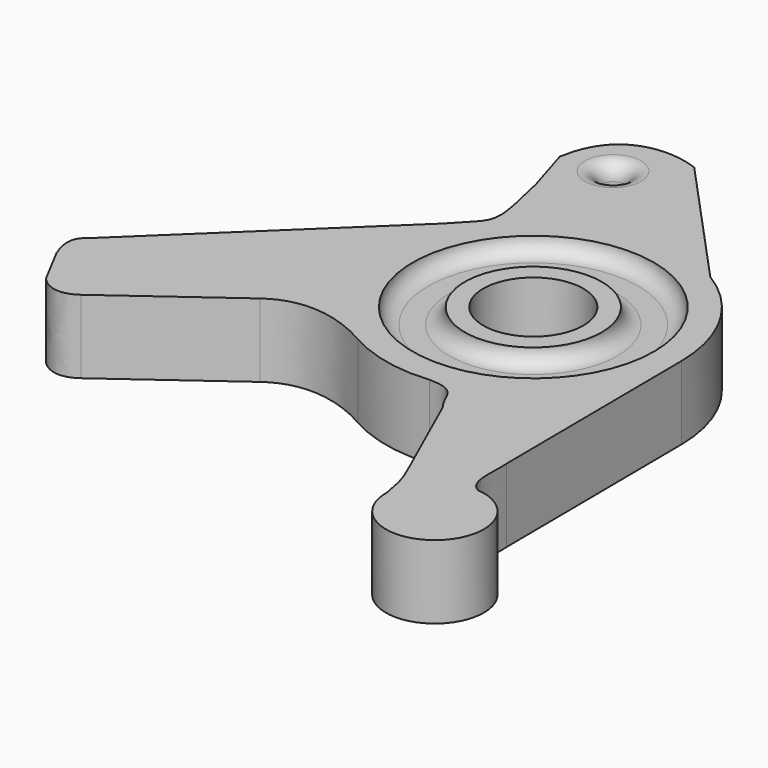
from build123d import *

# Parameters (mm, degrees)
F0_R     = 0.99695
F0_R_2   = 4.05765
F1_DEPTH = 5.9563
F2_R     = 9.7785511171
F2_R_2   = 5.5475367741
F3_DEPTH = 1.27
F4_R     = 1.26999
F5_R     = 1.27
F6_R     = 9.7785511171
F6_R_2   = 5.5475367741
F7_DEPTH = 1.27
F8_R     = 1.26999


# Not quite as in the source:
# - a fillet or chamfer is up to 0.001 mm smaller than in the source, because OpenCascade refuses the exact size


with BuildPart() as f1:
    # F0 (on Top) → F1 (new body)
    with BuildSketch(Plane.XY):
        with BuildLine():
            add(Edge.make_bspline(
                [(-33.6314394073, -33.2714746118), (-33.0057731764, -32.8335108579), (-30.3724482656, -30.8783296496), (-25.3025401745, -33.7471177082)],
                knots=[0, 0, 0, 0, 8.3424695855, 8.3424695855, 8.3424695855, 8.3424695855], degree=3))
            ThreePointArc((-25.3025401746, -33.7471177082), (-21.9177791625, -35.0471350698), (-18.2988837725, -35.2712966298))
            add(Edge.make_bspline(
                [(-18.2988837725, -35.2712966298), (-15.8398840576, -35.2424271405), (-16.2213556468, -36.5139991045), (-15.2587701461, -37.7152030189)],
                knots=[0, 0, 0, 0, 3.9006370377, 3.9006370377, 3.9006370377, 3.9006370377], degree=3))
            Line((-15.2587701461, -37.7152030189), (-11.9133347475, -45.1914166357))
            add(Edge.make_bspline(
                [(-10.7306365161, -49.0358446052), (-11.0024214771, -47.2270805733), (-11.3035654868, -46.5540988301), (-11.9133347475, -45.1914166357)],
                knots=[0, 0, 0, 0, 4.0222383717, 4.0222383717, 4.0222383717, 4.0222383717], degree=3))
            ThreePointArc((-10.7306365161, -49.0358446052), (-4.1177013069, -52.0873777347), (-6.4129489899, -45.1754601574))
            add(Edge.make_bspline(
                [(-6.4129489899, -45.1754601574), (-7.6786461286, -44.535394758), (-7.1622622199, -42.5141267478), (-7.293581398, -41.2180098819)],
                knots=[0, 0, 0, 0, 4.0542479106, 4.0542479106, 4.0542479106, 4.0542479106], degree=3))
            Line((-7.293581398, -41.2180098819), (-7.4388593588, -23.2832715275))
            ThreePointArc((-7.4388593588, -23.2832715275), (-9.004936212, -17.4677824297), (-13.2103104288, -13.1564789315))
            Line((-13.2103104288, -13.1564789315), (-23.3741309494, -2.0778968465))
            add(Edge.make_bspline(
                [(-30.9548836637, -6.2331505183), (-30.120029344, -0.9692255704), (-25.6342329085, -1.1884529376), (-23.3741309494, -2.0778968465)],
                knots=[0, 0, 0, 0, 8.6448796864, 8.6448796864, 8.6448796864, 8.6448796864], degree=3))
            Line((-30.9548836637, -6.2331505183), (-29.7779418645, -10.0919786303))
            add(Edge.make_bspline(
                [(-29.7779418645, -10.0919786303), (-28.2792598009, -16.4127741009), (-28.6187601862, -15.316130835), (-31.0345571488, -18.0451795459)],
                knots=[0, 0, 0, 0, 8.0518623173, 8.0518623173, 8.0518623173, 8.0518623173], degree=3))
            Line((-31.0345571488, -18.0451795459), (-47.0327663969, -33.3645439807))
            Line((-47.0327663969, -33.3645439807), (-47.710090224, -34.0131272307))
            add(Edge.make_bspline(
                [(-47.710090224, -34.0131272307), (-48.0070644447, -34.4292653886), (-48.1220479631, -35.0776240912), (-47.5788922065, -36.4427563472)],
                knots=[1.2296227613, 1.2296227613, 1.2296227613, 1.2296227613, 3.1262829004, 3.1262829004, 3.1262829004, 3.1262829004], degree=3))
            Line((-47.5788922065, -36.4427563472), (-45.9802214515, -39.4747166527))
            add(Edge.make_bspline(
                [(-45.9802214515, -39.4747166527), (-45.7317184979, -39.9460151291), (-44.362995404, -41.0978011232), (-42.7799038589, -39.9432815611)],
                knots=[0, 0, 0, 0, 3.234437473, 3.234437473, 3.234437473, 3.234437473], degree=3))
            Line((-42.7799038589, -39.9432815611), (-33.6314394073, -33.2714746118))
        make_face()
        with Locations((-27.0765330642, -5.6802984327)):
            Circle(F0_R, mode=Mode.SUBTRACT)
        with Locations((-19.3787027653, -23.3799886397)):
            Circle(F0_R_2, mode=Mode.SUBTRACT)
        with BuildLine():
            add(Edge.make_bspline(
                [(-47.0327663969, -33.3645439807), (-47.2485361779, -33.5711580997), (-47.5175590194, -33.7433409151), (-47.710090224, -34.0131272307)],
                knots=[0, 0, 0, 0, 1.2296227613, 1.2296227613, 1.2296227613, 1.2296227613], degree=3))
            Line((-47.710090224, -34.0131272307), (-47.0327663969, -33.3645439807))
        make_face()
    extrude(amount=F1_DEPTH)

    # F2 (on face) → F3 (cut)
    with BuildSketch(Plane.XY.offset(5.9563)):
        with Locations((-19.3787027653, -23.3799886397)):
            Circle(F2_R)
        with Locations((-19.3787027653, -23.3799886397)):
            Circle(F2_R_2, mode=Mode.SUBTRACT)
    extrude(amount=-F3_DEPTH, mode=Mode.SUBTRACT)

    # F4 (radius 1.27 in the source; OpenCascade refuses exactly that, so slightly less here)
    f4_edges = [f1.edges().sort_by_distance(p)[0] for p in [
        (-29.157254, -23.379989, 4.6863),
        (-24.92624, -23.379989, 4.6863),
    ]]
    fillet(f4_edges, radius=F4_R)

    # F5
    f5_edges = [f1.edges().sort_by_distance(p)[0] for p in [
        (-28.073483, -5.680298, 5.9563),
        (-28.073483, -5.680298, 0),
    ]]
    fillet(f5_edges, radius=F5_R)

    # F6 (on face) → F7 (cut)
    with BuildSketch(Plane(origin=(0, 0, 0), x_dir=(1, 0, 0), z_dir=(0, 0, -1))):
        with Locations((-19.3787027653, 23.3799886397)):
            Circle(F6_R)
        with Locations((-19.3787027653, 23.3799886397)):
            Circle(F6_R_2, mode=Mode.SUBTRACT)
    extrude(amount=-F7_DEPTH, mode=Mode.SUBTRACT)

    # F8 (radius 1.27 in the source; OpenCascade refuses exactly that, so slightly less here)
    f8_edges = [f1.edges().sort_by_distance(p)[0] for p in [
        (-29.157254, -23.379989, 1.27),
        (-24.92624, -23.379989, 1.27),
    ]]
    fillet(f8_edges, radius=F8_R)


solid = f1.part
